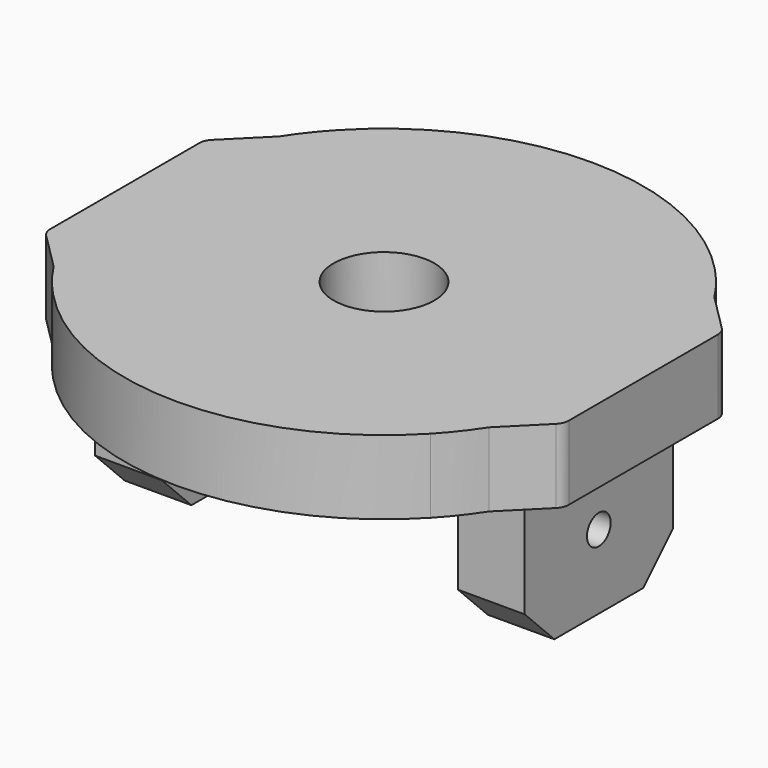
from build123d import *

# Parameters (mm, degrees)
F1_DEPTH      = 5
F3_SIZE       = 1
F2_W          = 4.5
F2_H          = 12.5
F4_DEPTH      = 10
F5_SIZE       = 2.5
F6_R          = 1
F7_DEPTH      = 39.5010001
F8_R          = 39.5864097355
F8_R_2        = 17.5
F9_DEPTH      = 25
F10_R         = 3.4
F11_DEPTH     = 25
F13_DEPTH     = 5
F14_T4_DEPTH  = 32.2598396724
F14_S5_R      = 17.5
F14_T6_DEPTH  = 18
F14_T10_DEPTH = 32.2598396724
F14_S11_R     = 17.5
F14_T12_DEPTH = 18
F14_T16_DEPTH = 32.2598396724
F14_S17_R     = 17.5
F14_T18_DEPTH = 18
F14_T22_DEPTH = 32.2598396724
F14_S23_R     = 17.5
F14_T24_DEPTH = 18
F15_R         = 1


# Not quite as in the source:
# - a fillet or chamfer that OpenCascade refuses, or shapes differently, is made with other operations: its cross-section is extruded or revolved along the edge and cut away or added


with BuildPart() as f1:
    # F0 (on Top) → F1 (new body)
    with BuildSketch(Plane.XY):
        with BuildLine():
            ThreePointArc((19.8625961196, -15.8301909188), (23.6080012184, -12.5093598908), (25, -7.7012087429))
            Line((25, -7.7012087429), (25, 7.7012087429))
            ThreePointArc((25, 7.7012087429), (23.6080012184, 12.5093598908), (19.8625961196, 15.8301909188))
            add(Edge.make_bspline(
                [(19.8625961196, 15.8301909188), (0, 25.2681728257), (-19.8625961196, 15.8301909188)],
                knots=[0.9132750433, 0.9132750433, 0.9132750433, 2.2283176103, 2.2283176103, 2.2283176103], degree=2, weights=[1, 0.7915095459, 1]))
            ThreePointArc((-19.8625961196, 15.8301909188), (-23.6080012184, 12.5093598908), (-25, 7.7012087429))
            Line((-25, 7.7012087429), (-25, -7.7012087429))
            ThreePointArc((-25, -7.7012087429), (-23.6080012184, -12.5093598908), (-19.8625961196, -15.8301909188))
            add(Edge.make_bspline(
                [(-19.8625961196, -15.8301909188), (0, -25.2681728257), (19.8625961196, -15.8301909188)],
                knots=[4.0548676969, 4.0548676969, 4.0548676969, 5.3699102639, 5.3699102639, 5.3699102639], degree=2, weights=[1, 0.7915095459, 1]))
        make_face()
    extrude(amount=F1_DEPTH)

    # F3
    f3_edges = [f1.edges().sort_by_distance(p)[0] for p in [
        (4e-06, -20, 0),
    ]]
    chamfer(f3_edges, length=F3_SIZE)

    # F2 (on face) → F4 (join)
    with BuildSketch(Plane(origin=(0, 0, 0), x_dir=(1, 0, 0), z_dir=(0, 0, -1))):
        with Locations((12.25, 0)):
            Rectangle(F2_W, F2_H)
        with Locations((-12.25, 0)):
            Rectangle(F2_W, F2_H)
    extrude(amount=F4_DEPTH)

    # F5
    f5_edges = [f1.edges().sort_by_distance(p)[0] for p in [
        (-12.25, -6.25, -10),
        (12.25, -6.25, -10),
        (-12.25, 6.25, -10),
        (12.25, 6.25, -10),
    ]]
    chamfer(f5_edges, length=F5_SIZE)

    # F6 (on face) → F7 (cut, through all)
    with BuildSketch(Plane.YZ.offset(14.5)):
        with Locations((0, -5)):
            Circle(F6_R)
    extrude(amount=-F7_DEPTH, mode=Mode.SUBTRACT)

    # F8 (on face) → F9 (cut)
    with BuildSketch(Plane.XY.offset(5)):
        Circle(F8_R)
        with BuildLine():
            add(Edge.make_bspline(
                [(-19.8625961196, -15.8301909188), (0, -25.2681728257), (19.8625961196, -15.8301909188)],
                knots=[4.0548676969, 4.0548676969, 4.0548676969, 5.3699102639, 5.3699102639, 5.3699102639], degree=2, weights=[1, 0.7915095459, 1]))
            ThreePointArc((-19.8625961196, -15.8301909188), (-23.6080012184, -12.5093598908), (-25, -7.7012087429))
            Line((-25, -7.7012087429), (-25, 7.7012087429))
            ThreePointArc((-25, 7.7012087429), (-23.6080012184, 12.5093598908), (-19.8625961196, 15.8301909188))
            add(Edge.make_bspline(
                [(19.8625961196, 15.8301909188), (0, 25.2681728257), (-19.8625961196, 15.8301909188)],
                knots=[0.9132750433, 0.9132750433, 0.9132750433, 2.2283176103, 2.2283176103, 2.2283176103], degree=2, weights=[1, 0.7915095459, 1]))
            ThreePointArc((19.8625961196, 15.8301909188), (23.6080012184, 12.5093598908), (25, 7.7012087429))
            Line((25, 7.7012087429), (25, -7.7012087429))
            ThreePointArc((25, -7.7012087429), (23.6080012184, -12.5093598908), (19.8625961196, -15.8301909188))
        make_face(mode=Mode.SUBTRACT)
        with BuildLine():
            ThreePointArc((-25, -7.7012087429), (-23.6080012184, -12.5093598908), (-19.8625961196, -15.8301909188))
            add(Edge.make_bspline(
                [(-19.8625961196, -15.8301909188), (0, -25.2681728257), (19.8625961196, -15.8301909188)],
                knots=[4.0548676969, 4.0548676969, 4.0548676969, 5.3699102639, 5.3699102639, 5.3699102639], degree=2, weights=[1, 0.7915095459, 1]))
            ThreePointArc((19.8625961196, -15.8301909188), (23.6080012184, -12.5093598908), (25, -7.7012087429))
            Line((25, -7.7012087429), (25, 7.7012087429))
            ThreePointArc((25, 7.7012087429), (23.6080012184, 12.5093598908), (19.8625961196, 15.8301909188))
            add(Edge.make_bspline(
                [(19.8625961196, 15.8301909188), (0, 25.2681728257), (-19.8625961196, 15.8301909188)],
                knots=[0.9132750433, 0.9132750433, 0.9132750433, 2.2283176103, 2.2283176103, 2.2283176103], degree=2, weights=[1, 0.7915095459, 1]))
            ThreePointArc((-19.8625961196, 15.8301909188), (-23.6080012184, 12.5093598908), (-25, 7.7012087429))
            Line((-25, 7.7012087429), (-25, -7.7012087429))
        make_face()
        Circle(F8_R_2, mode=Mode.SUBTRACT)
    extrude(amount=-F9_DEPTH, mode=Mode.SUBTRACT)

    # F10 (on face) → F11 (cut)
    with BuildSketch(Plane.XY.offset(5)):
        Circle(F10_R)
    extrude(amount=-F11_DEPTH, mode=Mode.SUBTRACT)

    # F12 (on face) → F13 (join)
    with BuildSketch(Plane(origin=(0, 0, 0), x_dir=(1, 0, 0), z_dir=(0, 0, -1))):
        with BuildLine():
            Line((-17.5, 12), (-17.5, -1.86e-08))
            ThreePointArc((-17.5, -1.86e-08), (-16.2659219885, 6.4552135413), (-12.7377392029, 12))
            Line((-12.7377392029, 12), (-17.5, 12))
        make_face()
        with BuildLine():
            ThreePointArc((12.7377392029, 12), (16.2659219851, 6.4552135499), (17.5, 0))
            Line((17.5, 0), (17.5, 12))
            Line((17.5, 12), (12.7377392029, 12))
        make_face()
        with BuildLine():
            Line((12.7377392029, -12), (17.5, -12))
            Line((17.5, -12), (17.5, 0))
            ThreePointArc((17.5, 0), (16.2659219851, -6.4552135499), (12.7377392029, -12))
        make_face()
        with BuildLine():
            Line((-17.5, -12), (-12.7377392029, -12))
            ThreePointArc((-12.7377392029, -12), (-16.2659219817, -6.4552135586), (-17.5, -1.86e-08))
            Line((-17.5, -1.86e-08), (-17.5, -12))
        make_face()
    extrude(amount=-F13_DEPTH)

    # F14: chamfer of 5.3 on 4 edges, made by hand


with BuildPart() as f14_tool2:
    # F14_s3 → F14_t4 (new body)
    with BuildSketch(Plane.XY.offset(-13.6299198362)):
        Polygon((17.5, -6.7), (12.2, -12), (17.5, -12), align=None)
    extrude(amount=F14_T4_DEPTH)

    # F14_s5 → F14_t6 (cut, symmetric)
    with BuildSketch(Plane.XY.offset(2.5)):
        Circle(F14_S5_R)
    extrude(amount=F14_T6_DEPTH, both=True, mode=Mode.SUBTRACT)


with BuildPart() as f1_1:
    add(f1.part)

    # F14_t1: cut F14_tool2
    add(f14_tool2.part, mode=Mode.SUBTRACT)


with BuildPart() as f14_tool8:
    # F14_s9 → F14_t10 (new body)
    with BuildSketch(Plane.XY.offset(-13.6299198362)):
        Polygon((12.2, 12), (17.5, 6.7), (17.5, 12), align=None)
    extrude(amount=F14_T10_DEPTH)

    # F14_s11 → F14_t12 (cut, symmetric)
    with BuildSketch(Plane.XY.offset(2.5)):
        Circle(F14_S11_R)
    extrude(amount=F14_T12_DEPTH, both=True, mode=Mode.SUBTRACT)


with BuildPart() as f1_2:
    add(f1_1.part)

    # F14_t7: cut F14_tool8
    add(f14_tool8.part, mode=Mode.SUBTRACT)


with BuildPart() as f14_tool14:
    # F14_s15 → F14_t16 (new body)
    with BuildSketch(Plane.XY.offset(-13.6299198362)):
        Polygon((-12.2, -12), (-17.5, -6.7), (-17.5, -12), align=None)
    extrude(amount=F14_T16_DEPTH)

    # F14_s17 → F14_t18 (cut, symmetric)
    with BuildSketch(Plane.XY.offset(2.5)):
        Circle(F14_S17_R)
    extrude(amount=F14_T18_DEPTH, both=True, mode=Mode.SUBTRACT)


with BuildPart() as f1_3:
    add(f1_2.part)

    # F14_t13: cut F14_tool14
    add(f14_tool14.part, mode=Mode.SUBTRACT)


with BuildPart() as f14_tool20:
    # F14_s21 → F14_t22 (new body)
    with BuildSketch(Plane.XY.offset(-13.6299198362)):
        Polygon((-17.5, 6.7), (-12.2, 12), (-17.5, 12), align=None)
    extrude(amount=F14_T22_DEPTH)

    # F14_s23 → F14_t24 (cut, symmetric)
    with BuildSketch(Plane.XY.offset(2.5)):
        Circle(F14_S23_R)
    extrude(amount=F14_T24_DEPTH, both=True, mode=Mode.SUBTRACT)


with BuildPart() as f1_4:
    add(f1_3.part)

    # F14_t19: cut F14_tool20
    add(f14_tool20.part, mode=Mode.SUBTRACT)

    # F15
    f15_edges = [f1_4.edges().sort_by_distance(p)[0] for p in [
        (-17.5, -6.7, 2.5),
        (-17.5, 6.7, 2.5),
        (17.5, 6.7, 2.5),
        (17.5, -6.7, 2.5),
    ]]
    fillet(f15_edges, radius=F15_R)


solid = f1_4.part
